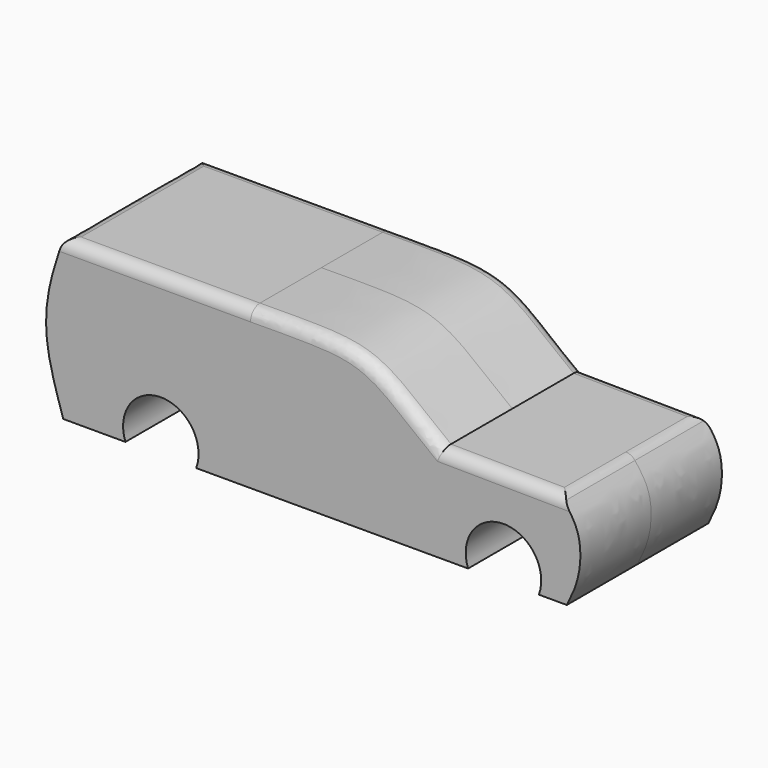
from build123d import *

# Parameters (mm, degrees)
F1_DEPTH = 19.05
F2_R     = 2.54


# Not quite as in the source:
# - a feature of the source that left no trace in its solid (it failed there, or was rolled back) is left out
# - the program builds the solid bodies; features that only make, move or delete a surface that nothing else refers to are left out


with BuildPart() as f1:
    # F0 (on Front) → F1 (new body, symmetric)
    with BuildSketch(Plane.XZ):
        with BuildLine():
            Line((57.1580786184, 0), (63.1808337388, 0))
            add(Edge.make_bspline(
                [(63.1808337388, 0), (64.1070753603, 1.8610503512), (66.0809264552, 5.8270093279), (66.4899415159, 14.6578153912), (63.3565966702, 18.5563140043), (61.8450880558, 20.4369286596)],
                knots=[0, 0, 0, 0, 0.3139594033, 0.669057725, 1, 1, 1, 1], degree=3))
            Line((61.8450880558, 20.4369286596), (36.198740513, 20.7040771047))
            add(Edge.make_bspline(
                [(36.198740513, 20.7040771047), (34.2669116908, 22.189306267), (29.9242250959, 25.5280517601), (20.2820782894, 33.6171914647), (6.7709379775, 34.1670870206), (-1.1152122764, 34.0960294227), (-4.942264819, 34.0615460371)],
                knots=[0, 0, 0, 0, 0.2093274169, 0.4705610335, 0.7430697263, 1, 1, 1, 1], degree=3))
            Line((-4.942264819, 34.0615460371), (-45.2818187647, 34.0615460371))
            add(Edge.make_bspline(
                [(-45.2818187647, 34.0615460371), (-46.4011998646, 30.7970228492), (-48.6607847814, 24.2072498428), (-49.5278252711, 13.2391089732), (-46.7579858308, 4.6027100105), (-45.2818187647, 0)],
                knots=[0, 0, 0, 0, 0.3143769013, 0.6346018389, 1, 1, 1, 1], degree=3))
            Line((-45.2818187647, 0), (-31.8846153722, 0))
            ThreePointArc((-31.8846153722, 0), (-24.2646153722, 10.9564242963), (-16.6446153722, 0))
            Line((-16.6446153722, 0), (41.9180786184, 0))
            ThreePointArc((41.9180786184, 0), (49.5380786184, 10.9564242963), (57.1580786184, 0))
        make_face()
    extrude(amount=F1_DEPTH, both=True)

    # F2
    f2_edges = [f1.edges().sort_by_distance(p)[0] for p in [
        (49.021914, -19.05, 20.570503),
        (49.021914, 19.05, 20.570503),
        (61.845088, 9.525, 20.436929),
        (61.845088, -9.525, 20.436929),
        (17.503149, -19.05, 32.967083),
        (17.503149, 19.05, 32.967083),
        (-45.281819, -9.525, 34.061546),
        (-45.281819, 9.525, 34.061546),
        (-25.112042, 19.05, 34.061546),
        (-25.112042, -19.05, 34.061546),
    ]]
    fillet(f2_edges, radius=F2_R)


solid = f1.part
